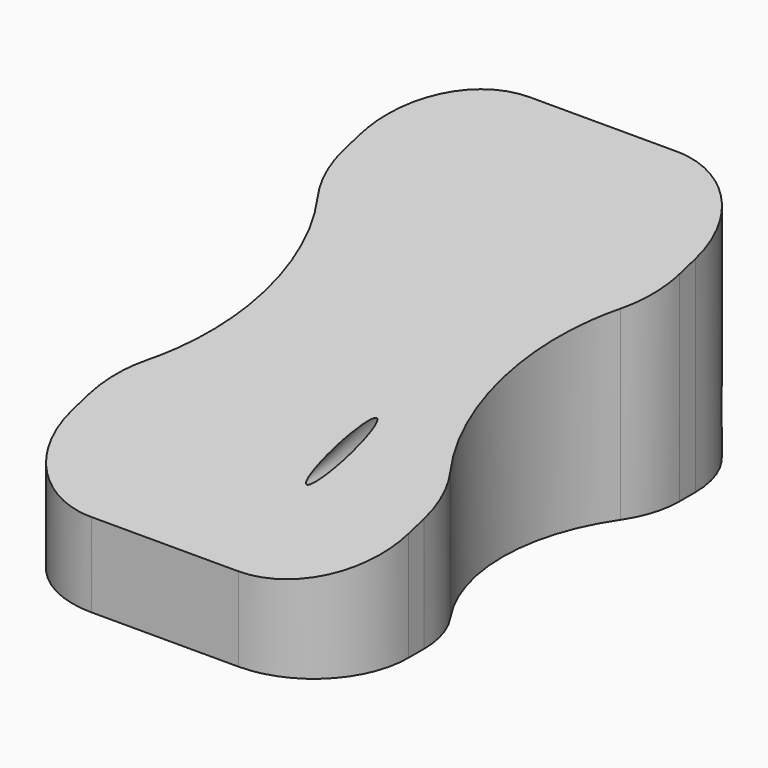
from build123d import *

# Parameters (mm, degrees)
F0_W     = 16
F0_H     = 26.1
F1_DEPTH = 11
F2_R     = 9
F3_DEPTH = 25
F5_DEPTH = 12.5
F6_R     = 4.5
F7_R     = 4.25


# Not quite as in the source:
# - an extrude whose draft closes it to a point is written as a loft to that point


with BuildPart() as f1:
    # F0 (on Top) → F1 (new body)
    with BuildSketch(Plane.XY):
        with Locations((0, 13.05)):
            Rectangle(F0_W, F0_H)
    extrude(amount=F1_DEPTH)

    # F2 (on Top) → F3 (cut)
    with BuildSketch(Plane.XY):
        with Locations((-14.65, 13.05)):
            Circle(F2_R)
        with Locations((14.65, 13.05)):
            Circle(F2_R)
    extrude(amount=F3_DEPTH, mode=Mode.SUBTRACT)

    # F4 (on Right) → F5 (cut, symmetric)
    with BuildSketch(Plane.YZ):
        Polygon((0, 4), (26.1, 11), (0, 11), align=None)
    extrude(amount=F5_DEPTH, both=True, mode=Mode.SUBTRACT)

    # F6
    f6_edges = [f1.edges().sort_by_distance(p)[0] for p in [
        (-8, 26.1, 5.5),
        (-8, 6.985554, 2.93676),
        (-8, 19.114446, 4.56324),
        (-8, 0, 2),
        (8, 0, 2),
        (8, 6.985554, 2.93676),
        (8, 19.114446, 4.56324),
        (8, 26.1, 5.5),
    ]]
    fillet(f6_edges, radius=F6_R)

    # F7 (on face) → F8 section 0
    with BuildSketch(Plane(origin=(0, 26.1, 0), x_dir=(-1, 0, 0), z_dir=(0, 1, 0)), mode=Mode.PRIVATE) as f8_s0:
        with Locations((-2.75, 5.5)):
            Circle(F7_R)
    loft([f8_s0.sketch, Vertex(2.75, 4.2356454321, 5.5)], ruled=True, mode=Mode.SUBTRACT)


solid = f1.part
